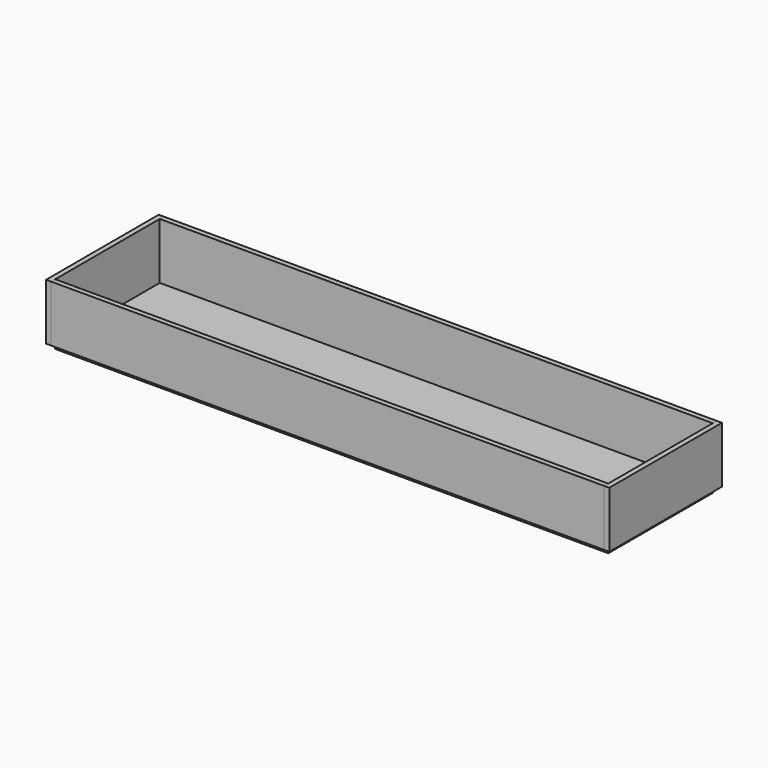
from build123d import *

# Parameters (mm, degrees)
F1_DEPTH = 200
F0_W     = 1964
F0_H     = 18
F2_DEPTH = 200
F0_H_2   = 464
F3_DEPTH = 18


# Not quite as in the source:
# - the program builds the solid bodies; features that only make, move or delete a surface that nothing else refers to are left out


with BuildPart() as f1:
    # F0 (on Top) → F1 (new body)
    with BuildSketch(Plane.XY):
        Polygon((-1923.9414028525, 431.0778304935), (-1941.9414028525, 431.0778304935), (-1941.9414028525, -68.9221695065), (-1923.9414028525, -68.9221695065), (-1923.9414028525, -50.9221695065), (-1923.9414028525, 413.0778304935), align=None)
    extrude(amount=F1_DEPTH)


with BuildPart() as f1b:
    # F0 (on Top) → F1, piece 2 (new body)
    with BuildSketch(Plane.XY):
        Polygon((58.0585971475, 431.0778304935), (40.0585971475, 431.0778304935), (40.0585971475, 413.0778304935), (40.0585971475, -50.9221695065), (40.0585971475, -68.9221695065), (58.0585971475, -68.9221695065), align=None)
    extrude(amount=F1_DEPTH)


with BuildPart() as f2:
    # F0 (on Top) → F2 (new body)
    with BuildSketch(Plane.XY):
        with Locations((-941.9414028525, 422.0778304935)):
            Rectangle(F0_W, F0_H)
    extrude(amount=F2_DEPTH)


with BuildPart() as f2b:
    # F0 (on Top) → F2, piece 2 (new body)
    with BuildSketch(Plane.XY):
        with Locations((-941.9414028525, -59.9221695065)):
            Rectangle(F0_W, F0_H)
    extrude(amount=F2_DEPTH)


with BuildPart() as f3:
    # F0 (on Top) → F3 (new body)
    with BuildSketch(Plane.XY):
        with Locations((-941.9414028525, 181.0778304935)):
            Rectangle(F0_W, F0_H_2)
    extrude(amount=-F3_DEPTH)


solid = Compound([f1.part, f1b.part, f2.part, f2b.part, f3.part])
